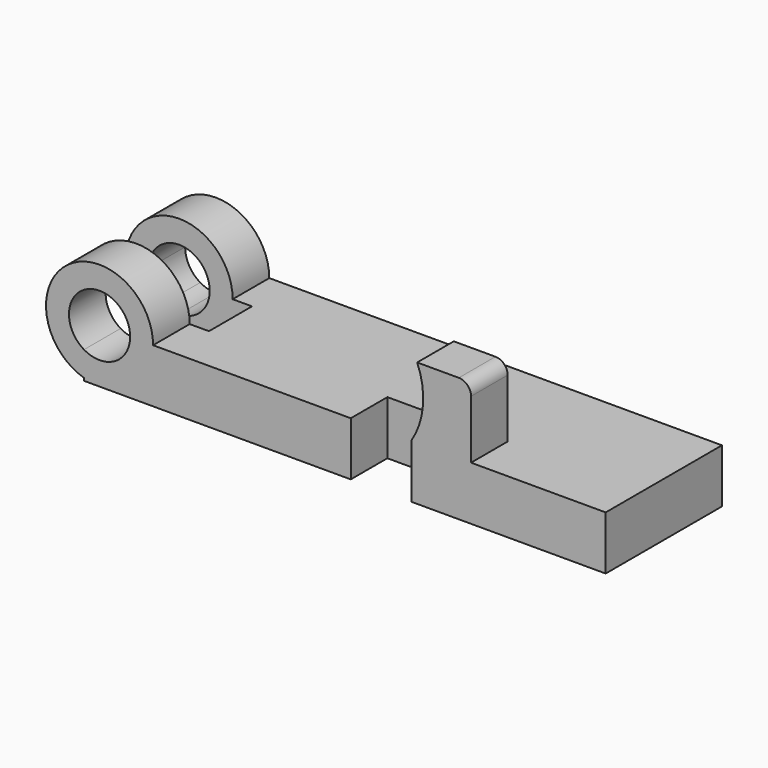
from build123d import *
from build123d import SkipClean  # not in build123d's __all__

# Parameters (mm, degrees)
F1_DEPTH = 22.352
F4_DEPTH = 60.326
F5_DEPTH = 18.9992
F6_DEPTH = 18.9992
F8_DEPTH = 18.9992


with BuildPart() as f1:
    # F0 (on Top) → F1 (new body)
    with BuildSketch(Plane.XY):
        Polygon((105.8206515543, 17.5817109668), (-110.7397484457, 17.5817109668), (-110.7397484457, -1.4174890332), (-74.0668755353, -1.4174890332), (-74.0668755353, -23.7440890332), (-110.7397484457, -23.7440890332), (-110.7397484457, -42.7432890332), (0, -42.7432890332), (0, -23.7440890332), (25.1433271915, -23.7440890332), (25.1433271915, -42.7432890332), (105.8206515543, -42.7432890332), align=None)
    extrude(amount=F1_DEPTH)

    # F2 (on face) → F4 (cut, through all)
    with BuildSketch(Plane.XZ.offset(42.7432890332)):
        with BuildLine():
            ThreePointArc((-110.7397484457, 11.4130391755), (-97.9889229317, 11.3240532527), (-91.5876839638, 22.352))
            Line((-91.5876839638, 22.352), (-110.7397484457, 22.352))
            Line((-110.7397484457, 22.352), (-110.7397484457, 11.4130391755))
        make_face()
    extrude(amount=-F4_DEPTH, mode=Mode.SUBTRACT)

    # F2 (on face) → F5 (join)
    with BuildSketch(Plane.XZ.offset(42.7432890332)):
        with BuildLine():
            ThreePointArc((-110.7397484457, 1.0841489351), (-91.0484715271, 4.5005608688), (-82.0626839638, 22.352))
            Line((-82.0626839638, 22.352), (-91.5876839638, 22.352))
            ThreePointArc((-91.5876839638, 22.352), (-97.9889229317, 11.3240532527), (-110.7397484457, 11.4130391755))
            Line((-110.7397484457, 11.4130391755), (-110.7397484457, 1.0841489351))
        make_face()
        with BuildLine():
            Line((-91.5876839638, 22.352), (-82.0626839638, 22.352))
            ThreePointArc((-82.0626839638, 22.352), (-117.5268964005, 40.2034391312), (-110.7397484457, 1.0841489351))
            Line((-110.7397484457, 1.0841489351), (-110.7397484457, 11.4130391755))
            ThreePointArc((-110.7397484457, 11.4130391755), (-110.5864449959, 33.3799467473), (-91.5876839638, 22.352))
        make_face()
    with SkipClean():  # cleaning this boolean's faces spoils the solid; the shape is the same uncleaned
        extrude(amount=-F5_DEPTH)

    # F3 (on face) → F6 (join)
    with BuildSketch(Plane(origin=(0, 17.5817109668, 0), x_dir=(-1, 0, 0), z_dir=(0, 1, 0))):
        with BuildLine():
            Line((91.6125912547, 22.352), (82.0875912547, 22.352))
            ThreePointArc((82.0875912547, 22.352), (91.062929817, 4.5083149326), (110.7397484457, 1.0766086889))
            Line((110.7397484457, 1.0766086889), (110.7397484457, 11.3983864208))
            ThreePointArc((110.7397484457, 11.3983864208), (98.0012877573, 11.331226517), (91.6125912547, 22.352))
        make_face()
        with BuildLine():
            ThreePointArc((110.7397484457, 1.0766086889), (122.1562763221, 9.1023385623), (126.5375912547, 22.352))
            ThreePointArc((126.5375912547, 22.352), (104.3125912547, 44.577), (82.0875912547, 22.352))
            Line((82.0875912547, 22.352), (91.6125912547, 22.352))
            ThreePointArc((91.6125912547, 22.352), (104.3125912547, 35.052), (117.0125912547, 22.352))
            ThreePointArc((117.0125912547, 22.352), (115.3333647377, 16.0406965025), (110.7397484457, 11.3983864208))
            Line((110.7397484457, 11.3983864208), (110.7397484457, 1.0766086889))
        make_face()
    extrude(amount=-F6_DEPTH)

    # F7 (on face) → F8 (join)
    with BuildSketch(Plane.XZ.offset(42.7432890332)):
        with BuildLine():
            Line((44.8509039521, 51.7072044313), (27.5659821928, 51.7072044313))
            ThreePointArc((27.5659821928, 51.7072044313), (29.9657018108, 36.7315861898), (25.1433271915, 22.352))
            Line((25.1433271915, 22.352), (49.9309039521, 22.352))
            Line((49.9309039521, 22.352), (49.9309039521, 46.6272044313))
            ThreePointArc((49.9309039521, 46.6272044313), (48.4430064005, 50.2193068797), (44.8509039521, 51.7072044313))
        make_face()
    extrude(amount=-F8_DEPTH)


solid = f1.part
